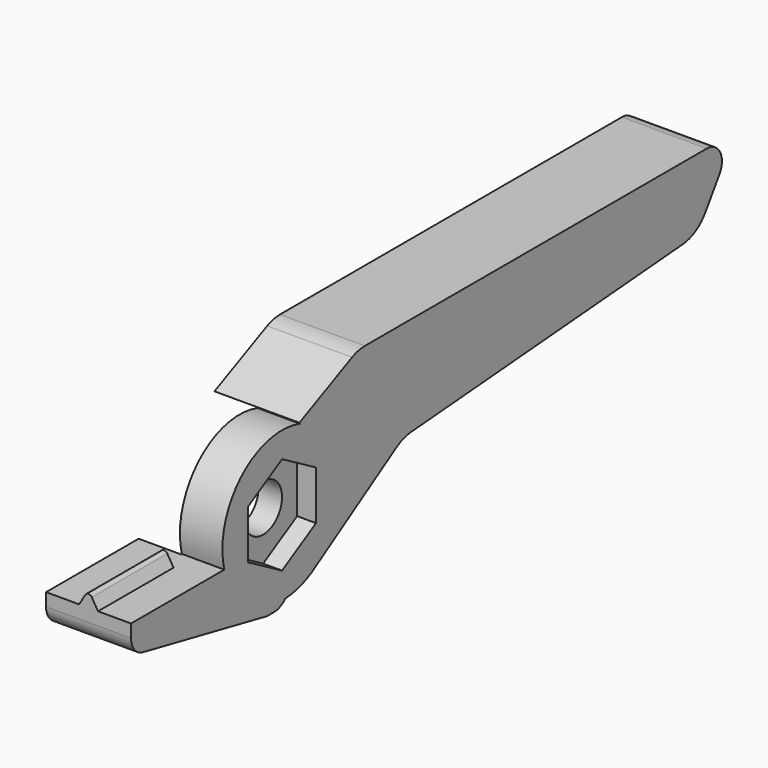
from build123d import *

# Parameters (mm, degrees)
F2_DEPTH     = 5.715
F3_R         = 5.08
F4_R         = 2.54
F0_R         = 3.175
F5_DEPTH     = 5.715
F7_DEPTH     = 25.4
F9_DEPTH     = 5.715
F10_T1_DEPTH = 10.4031462071
F10_T3_DEPTH = 10.4031460084
F10_T5_DEPTH = 21.8251062119
F12_DEPTH    = 12.7
F13_R        = 0.508
F15_DEPTH    = 2.54


# Not quite as in the source:
# - a fillet or chamfer that OpenCascade refuses, or shapes differently, is made with other operations: its cross-section is extruded or revolved along the edge and cut away or added


with BuildPart() as f2:
    # F1 (on Right) → F2 (new body, symmetric)
    with BuildSketch(Plane.YZ):
        Polygon((20.3924354673, 0.8880047341), (69.85, 4.8502287827), (76.2, 14.35636729), (12.8064267337, 14.35636729), (2.9200423986, 9.7313386741), (8.2383593544, 1.7451149179), (4.8682624474, -6.6303843632), (5.9557488763, -8.2313216024), align=None)
    extrude(amount=F2_DEPTH, both=True)

    # F3
    f3_edges = [f2.edges().sort_by_distance(p)[0] for p in [
        (0, 12.806427, 14.356367),
        (0, 69.85, 4.850229),
        (0, 20.392435, 0.888005),
    ]]
    fillet(f3_edges, radius=F3_R)

    # F4
    f4_edges = [f2.edges().sort_by_distance(p)[0] for p in [
        (0, 76.2, 14.356367),
    ]]
    fillet(f4_edges, radius=F4_R)

    # F0 (on Right) → F5 (join)
    with BuildSketch(Plane.YZ):
        with BuildLine():
            Line((10.16, 0), (10.033, 0))
            ThreePointArc((10.033, 0), (-1.2804712188, 9.9509538466), (-9.7061572726, -2.54))
            Line((-9.7061572726, -2.54), (-9.8373776994, -2.54))
            ThreePointArc((-9.8373776994, -2.54), (1.2802036116, -10.0790217141), (10.16, 0))
        make_face()
        Circle(F0_R, mode=Mode.SUBTRACT)
    extrude(amount=F5_DEPTH)

    # F6 (on Right) → F7 (cut)
    with BuildSketch(Plane.YZ):
        with BuildLine():
            Line((19.0573167056, 0), (5.4165862694, 8.5957078351))
            ThreePointArc((5.4165862694, 8.5957078351), (-10.1595718617, -0.0932715764), (5.5734885208, -8.4948116935))
            Line((5.5734885208, -8.4948116935), (19.0573167056, 0))
        make_face()
    extrude(amount=-F7_DEPTH, mode=Mode.SUBTRACT)

    # F8 (on Right) → F9 (join, symmetric)
    with BuildSketch(Plane.YZ):
        with BuildLine():
            Line((0.5413664183, -10.9723807834), (0.5413664183, -10.1455666378))
            ThreePointArc((0.5413664183, -10.1455666378), (-6.0054239987, -8.1951499434), (-9.8373776994, -2.54))
            Line((-9.8373776994, -2.54), (-25.4, -2.54))
            Line((-25.4, -2.54), (-25.4, -6.360667292))
            Line((-25.4, -6.360667292), (-2.5253696451, -10.9723807834))
            Line((-2.5253696451, -10.9723807834), (0.5413664183, -10.9723807834))
        make_face()
    extrude(amount=F9_DEPTH, both=True)

    # F10: fillet of radius 2.54 on 2 edges, made by hand

    # F10_s2 → F10_t1 (cut)
    with BuildSketch(Plane.YZ.offset(-10.4031461077)):
        with BuildLine():
            ThreePointArc((0.5413664183, -10.1455666378), (-0.3091706163, -10.7565034211), (-1.3338920247, -10.9723807834))
            Line((-1.3338920247, -10.9723807834), (0.5413664183, -10.9723807834))
            Line((0.5413664183, -10.9723807834), (0.5413664183, -10.1455666378))
        make_face()
    extrude(amount=F10_T1_DEPTH, mode=Mode.SUBTRACT)

    # F10_s4 → F10_t3 (cut)
    with BuildSketch(Plane.YZ.offset(9.94e-08)):
        with BuildLine():
            ThreePointArc((0.5413664183, -10.1455666378), (-0.3091706163, -10.7565034211), (-1.3338920247, -10.9723807834))
            Line((-1.3338920247, -10.9723807834), (0.5413664183, -10.9723807834))
            Line((0.5413664183, -10.9723807834), (0.5413664183, -10.1455666378))
        make_face()
    extrude(amount=F10_T3_DEPTH, mode=Mode.SUBTRACT)

    # F10_s6 → F10_t5 (cut)
    with BuildSketch(Plane.YZ.offset(-10.912553106)):
        with BuildLine():
            ThreePointArc((-23.3619846843, -6.7715479306), (-24.8255331463, -5.8904591062), (-25.4, -4.2816460496))
            Line((-25.4, -4.2816460496), (-25.4, -6.360667292))
            Line((-25.4, -6.360667292), (-23.3619846843, -6.7715479306))
        make_face()
    extrude(amount=F10_T5_DEPTH, mode=Mode.SUBTRACT)

    # F11 (on face) → F12 (join)
    with BuildSketch(Plane.XZ.offset(25.4)):
        Polygon((0, -0.4141342943), (-1.27, -2.54), (1.27, -2.54), align=None)
    extrude(amount=-F12_DEPTH)

    # F13
    f13_edges = [f2.edges().sort_by_distance(p)[0] for p in [
        (0, -19.05, -0.414134),
    ]]
    fillet(f13_edges, radius=F13_R)

    # F14 (on face) → F15 (cut)
    with BuildSketch(Plane.YZ.offset(5.715)):
        Polygon((5.715, -3.2995567884), (5.715, 3.2995567884), (0, 6.5991135768), (-5.715, 3.2995567884), (-5.715, -3.2995567884), (0, -6.5991135768), align=None)
    extrude(amount=-F15_DEPTH, mode=Mode.SUBTRACT)


solid = f2.part
